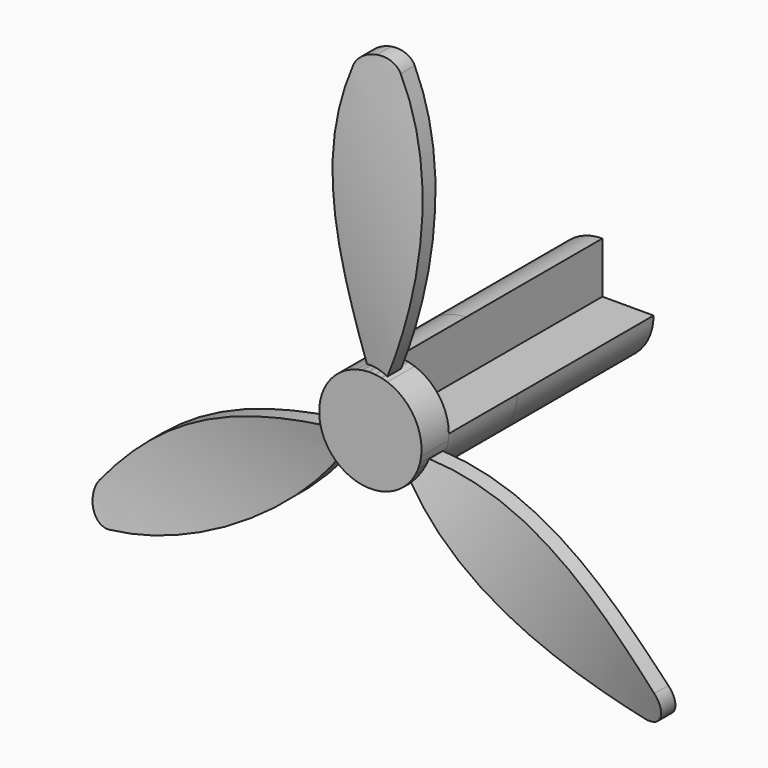
from build123d import *
from build123d import SkipClean  # not in build123d's __all__

# Parameters (mm, degrees)
F5_DEPTH  = 10
F6_R      = 15
F7_DEPTH  = 5
F8_COUNT  = 3
F9_DEPTH  = 25
F11_DEPTH = 50
F13_DEPTH = 85.0010001


# Not quite as in the source:
# - after a boolean that leaves OpenCascade's solid faulty, fix() repairs it


with BuildPart() as f3:
    # F1 (on Top) → F3 section 0
    with BuildSketch(Plane.XY):
        Polygon((24.347365878, -6.2012720312), (-22.6372651613, 10.8997351351), (-24.347365878, 6.2012720312), (22.6372651613, -10.8997351351), align=None)
    # F2 (on offset) → F3 section 1
    with BuildSketch(Plane.XY.offset(100)):
        Polygon((22.6372651613, 10.8997351351), (-24.347365878, -6.2012720312), (-22.6372651613, -10.8997351351), (24.347365878, 6.2012720312), align=None)
    loft()

    # F4 (on Front) → F5 (intersect, symmetric)
    with BuildSketch(Plane.XZ):
        with BuildLine():
            ThreePointArc((-5.5815786476, 92.201358626), (-12.3413751679, 48.9750162147), (0, 7))
            ThreePointArc((0, 7), (12.3413751679, 48.9750162147), (5.5815786476, 92.201358626))
            ThreePointArc((5.5815786476, 92.201358626), (3.3757849638, 94.9602495782), (0, 96))
            ThreePointArc((0, 96), (-3.3757849638, 94.9602495782), (-5.5815786476, 92.201358626))
        make_face()
    extrude(amount=F5_DEPTH, both=True, mode=Mode.INTERSECT)

    # F6 (on Front) → F7 (join, symmetric)
    with BuildSketch(Plane.XZ):
        Circle(F6_R)
    extrude(amount=F7_DEPTH, both=True)


with BuildPart() as f8_1:
    # F8: instance of F3
    add(f3.part.rotate(Axis((0, 0, 0), (0, -1, 0)), 1 * 360 / F8_COUNT), clean=False)


with BuildPart() as f8_2:
    # F8: instance of F3
    add(f3.part.rotate(Axis((0, 0, 0), (0, -1, 0)), 2 * 360 / F8_COUNT), clean=False)


with BuildPart() as f9:
    # F9 (new): a face of the model
    f9_faces = [f8_1.part.faces().sort_by_distance(p)[0] for p in [
        (0, 5, 0),
    ]]
    extrude(f9_faces, amount=F9_DEPTH)

    # F10 (on face) → F11 (join)
    with BuildSketch(Plane(origin=(0, 30, 0), x_dir=(-1, 0, 0), z_dir=(0, 1, 0))):
        with BuildLine():
            Line((0, 15), (0, 0))
            Line((0, 0), (12.8746125847, 0))
            Line((12.8746125847, 0), (12.8746125847, 7.697035195))
            ThreePointArc((12.8746125847, 7.697035195), (7.4008267131, 13.0471362361), (0, 15))
        make_face()
        with BuildLine():
            Line((12.8746125847, 0), (0, 0))
            Line((0, 0), (0, 15))
            ThreePointArc((0, 15), (-10.6066017178, -10.6066017178), (15, 0))
            ThreePointArc((15, 0), (14.4588932628, 3.9925437524), (12.8746125847, 7.697035195))
            Line((12.8746125847, 7.697035195), (12.8746125847, 0))
        make_face()
    with SkipClean():  # cleaning this boolean's faces spoils the solid; the shape is the same uncleaned
        extrude(amount=F11_DEPTH)

    # F12 (on face) → F13 (cut, through all)
    with BuildSketch(Plane(origin=(0, 80, 0), x_dir=(-1, 0, 0), z_dir=(0, 1, 0))):
        with BuildLine():
            Line((-15, 0), (0, 0))
            Line((0, 0), (0, 15))
            ThreePointArc((0, 15), (-10.6066017178, 10.6066017178), (-15, 0))
        make_face()
    extrude(amount=-F13_DEPTH, mode=Mode.SUBTRACT)

    add(f9.part.fix(), mode=Mode.REPLACE)


solid = Compound([f3.part, f8_1.part, f8_2.part, f9.part])
